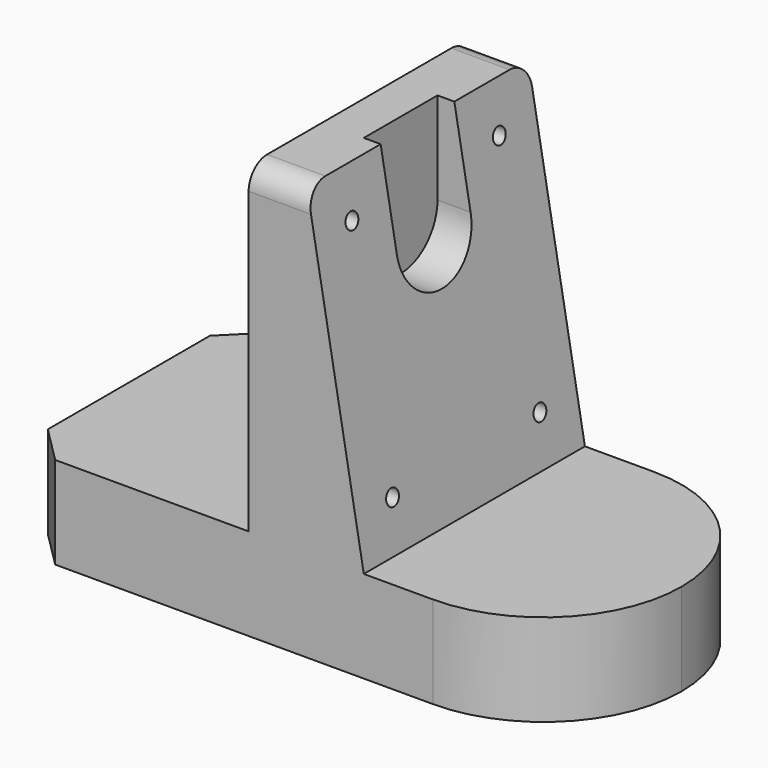
from build123d import *

# Parameters (mm, degrees)
F0_W           = 120
F0_H           = 60
F1_DEPTH       = 90
F2_W           = 50
F2_H           = 70
F2_W_2         = 45
F3_DEPTH       = 60.001
F4_R           = 29.99999
F5_SIZE        = 8
F7_D           = 3.4
F7_CBORE_D     = 7
F7_CBORE_DEPTH = 2.4
F9_DEPTH       = 16
F11_DEPTH      = 60.001
F12_R          = 5


# Not quite as in the source:
# - a fillet or chamfer is up to 0.001 mm smaller than in the source, because OpenCascade refuses the exact size


with BuildPart() as f1:
    # F0 (on Top) → F1 (new body)
    with BuildSketch(Plane.XY):
        with Locations((60, 30)):
            Rectangle(F0_W, F0_H)
    extrude(amount=F1_DEPTH)

    # F2 (on face) → F3 (cut, through all)
    with BuildSketch(Plane.XZ):
        with Locations((25, 55)):
            Rectangle(F2_W, F2_H)
        with Locations((97.5, 55)):
            Rectangle(F2_W_2, F2_H)
    extrude(amount=-F3_DEPTH, mode=Mode.SUBTRACT)

    # F4 (radius 30 in the source; OpenCascade refuses exactly that, so slightly less here)
    f4_edges = [f1.edges().sort_by_distance(p)[0] for p in [
        (120, 60, 10),
        (120, 0, 10),
    ]]
    fillet(f4_edges, radius=F4_R)

    # F5
    f5_edges = [f1.edges().sort_by_distance(p)[0] for p in [
        (0, 60, 10),
        (0, 0, 10),
    ]]
    chamfer(f5_edges, length=F5_SIZE)

    # F7 (through all)
    with Locations(Plane(origin=(50, 0, 0), x_dir=(0, -1, 0), z_dir=(-1, 0, 0))):
        with Locations((-50, 80), (-10, 80), (-10, 30), (-50, 30)):
            CounterBoreHole(F7_D / 2, F7_CBORE_D / 2, F7_CBORE_DEPTH)

    # F8 (on face) → F9 (cut)
    with BuildSketch(Plane.YZ.offset(75)):
        with BuildLine():
            Line((40, 90), (20, 90))
            Line((20, 90), (20, 70))
            ThreePointArc((20, 70), (30, 80), (40, 70))
            Line((40, 70), (40, 90))
        make_face()
        with BuildLine():
            ThreePointArc((40, 70), (30, 80), (20, 70))
            Line((20, 70), (40, 70))
        make_face()
        with BuildLine():
            Line((40, 70), (20, 70))
            ThreePointArc((20, 70), (30, 60), (40, 70))
        make_face()
    extrude(amount=-F9_DEPTH, mode=Mode.SUBTRACT)

    # F10 (on face) → F11 (cut, through all)
    with BuildSketch(Plane.XZ):
        Polygon((62.6571113504, 90), (75, 20), (75, 90), align=None)
    extrude(amount=-F11_DEPTH, mode=Mode.SUBTRACT)

    # F12
    f12_edges = [f1.edges().sort_by_distance(p)[0] for p in [
        (56.328556, 60, 90),
        (56.328556, 0, 90),
    ]]
    fillet(f12_edges, radius=F12_R)


solid = f1.part
